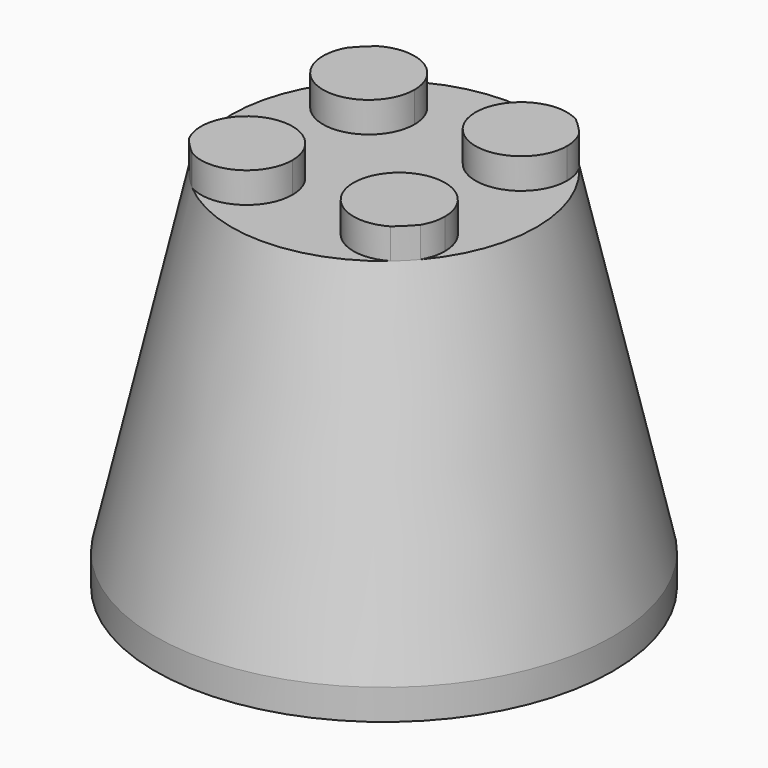
from build123d import *

# Parameters (mm, degrees)
F0_W     = 1.5875
F0_H     = 1.5875
F3_DEPTH = 1.5875
F4_R     = 3.175
F4_R_2   = 2.38125
F5_DEPTH = 1.5875


with BuildPart() as f1:
    # F0 (on Front) → F1 (revolve)
    with BuildSketch(Plane.XZ):
        with Locations((11.1125, 0.79375)):
            Rectangle(F0_W, F0_H)
        Polygon((0, 19.05), (0, 1.5875), (10.31875, 1.5875), (11.90625, 1.5875), (7.9375, 19.05), align=None)
    revolve(axis=Axis((0, 0, 9.525), (0, 0, 1)))

    # F2 (on face) → F3 (join)
    with BuildSketch(Plane.XY.offset(19.05)):
        with BuildLine():
            ThreePointArc((6.028877012, 5.162997988), (5.6126600757, 5.6126600757), (5.162997988, 6.028877012))
            ThreePointArc((5.162997988, 6.028877012), (1.9054814058, 2.7799378741), (6.35, 3.96875))
            ThreePointArc((6.35, 3.96875), (6.2683183301, 4.5870840986), (6.028877012, 5.162997988))
        make_face()
        with BuildLine():
            ThreePointArc((-1.5875, 3.96875), (-2.7799378741, 6.0320185942), (-5.162997988, 6.028877012))
            ThreePointArc((-5.162997988, 6.028877012), (-5.6126600757, 5.6126600757), (-6.028877012, 5.162997988))
            ThreePointArc((-6.028877012, 5.162997988), (-4.5870840986, 1.6691816699), (-1.5875, 3.96875))
        make_face()
        with BuildLine():
            ThreePointArc((-6.028877012, -5.162997988), (-5.6126600757, -5.6126600757), (-5.162997988, -6.028877012))
            ThreePointArc((-5.162997988, -6.028877012), (-2.7799378741, -6.0320185942), (-1.5875, -3.96875))
            ThreePointArc((-1.5875, -3.96875), (-4.5870840986, -1.6691816699), (-6.028877012, -5.162997988))
        make_face()
        with BuildLine():
            ThreePointArc((6.35, -3.96875), (1.9054814058, -2.7799378741), (5.162997988, -6.028877012))
            ThreePointArc((5.162997988, -6.028877012), (5.6126600757, -5.6126600757), (6.028877012, -5.162997988))
            ThreePointArc((6.028877012, -5.162997988), (6.2683183301, -4.5870840986), (6.35, -3.96875))
        make_face()
    extrude(amount=F3_DEPTH)

    # F4 (on face) → F5 (join)
    with BuildSketch(Plane(origin=(0, 0, 1.5875), x_dir=(1, 0, 0), z_dir=(0, 0, -1))):
        with Locations((-4.7625, -4.7625)):
            Circle(F4_R)
        with Locations((-4.7625, -4.7625)):
            Circle(F4_R_2, mode=Mode.SUBTRACT)
        with Locations((-4.7625, 4.7625)):
            Circle(F4_R)
        with Locations((-4.7625, 4.7625)):
            Circle(F4_R_2, mode=Mode.SUBTRACT)
        with Locations((4.7625, -4.7625)):
            Circle(F4_R)
        with Locations((4.7625, -4.7625)):
            Circle(F4_R_2, mode=Mode.SUBTRACT)
        with Locations((4.7625, 4.7625)):
            Circle(F4_R)
        with Locations((4.7625, 4.7625)):
            Circle(F4_R_2, mode=Mode.SUBTRACT)
    extrude(amount=F5_DEPTH)


solid = f1.part
